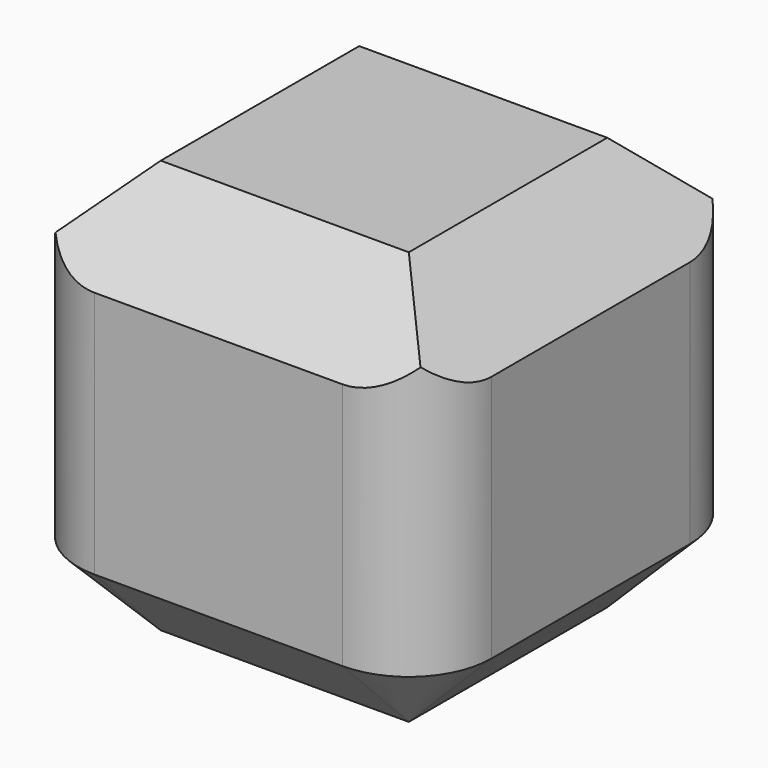
from build123d import *

# Parameters (mm, degrees)
F0_W     = 25.4
F0_H     = 25.4
F1_DEPTH = 25.4
F2_SIZE  = 5.08
F3_R     = 5.08
F4_SIZE  = 5.07999


# Not quite as in the source:
# - a fillet or chamfer is up to 0.001 mm smaller than in the source, because OpenCascade refuses the exact size


with BuildPart() as f1:
    # F0 (on Front) → F1 (new body)
    with BuildSketch(Plane.XZ):
        with Locations((12.7, 12.7)):
            Rectangle(F0_W, F0_H)
    extrude(amount=F1_DEPTH)

    # F2
    f2_edges = [f1.edges().sort_by_distance(p)[0] for p in [
        (25.4, -12.7, 25.4),
        (12.7, -25.4, 25.4),
        (12.7, 0, 25.4),
        (0, -12.7, 25.4),
    ]]
    chamfer(f2_edges, length=F2_SIZE)

    # F3
    f3_edges = [f1.edges().sort_by_distance(p)[0] for p in [
        (25.4, -25.4, 10.16),
        (25.4, 0, 10.16),
        (0, -25.4, 10.16),
        (0, 0, 10.16),
    ]]
    fillet(f3_edges, radius=F3_R)

    # F4 (size 5.08 in the source; OpenCascade refuses exactly that, so slightly less here)
    f4_edges = [f1.edges().sort_by_distance(p)[0] for p in [
        (12.7, -25.4, 0),
    ]]
    chamfer(f4_edges, length=F4_SIZE)


solid = f1.part
